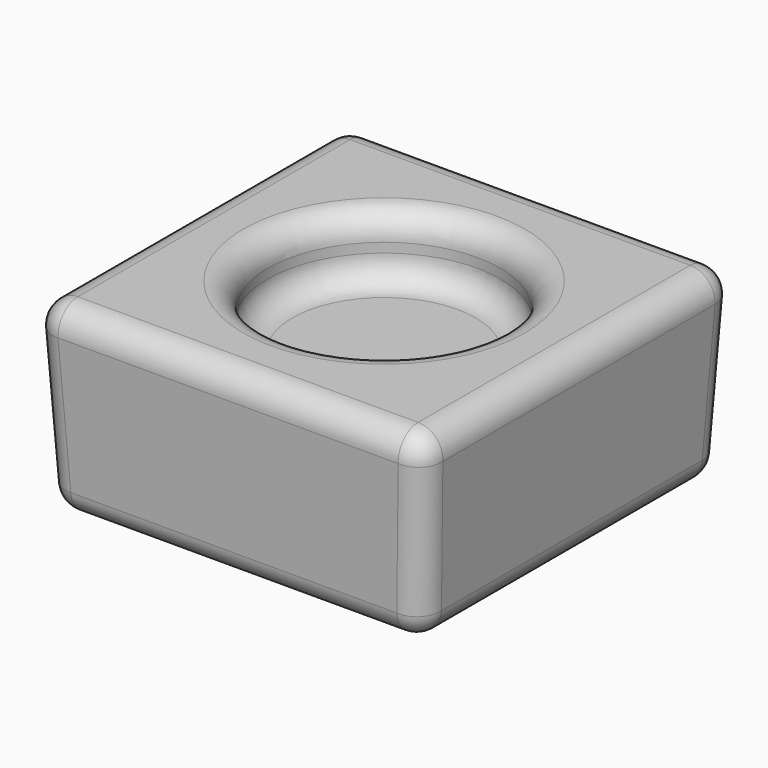
from build123d import *

# Parameters (mm, degrees)
F0_W     = 30
F0_H     = 30
F0_R     = 10
F1_DEPTH = 15
F1_TAPER = -3
F2_DEPTH = 10
F3_R     = 2


with BuildPart() as f1:
    # F0 (on Top) → F1 (new body)
    with BuildSketch(Plane.XY):
        with Locations((-58.3209823817, -55.5250146758)):
            Rectangle(F0_W, F0_H)
        with Locations((-58.3209823817, -55.5250146758)):
            Circle(F0_R, mode=Mode.SUBTRACT)
    extrude(amount=F1_DEPTH, taper=F1_TAPER)

    # F0 (on Top) → F2 (join)
    with BuildSketch(Plane.XY):
        with Locations((-58.3209823817, -55.5250146758)):
            Circle(F0_R)
    extrude(amount=F2_DEPTH)

    # F3
    f3_edges = [f1.edges().sort_by_distance(p)[0] for p in [
        (-67.796905, -55.525015, 10),
        (-67.534866, -55.525015, 15),
        (-42.534866, -55.525015, 15),
        (-58.320982, -39.738898, 15),
        (-58.320982, -71.311131, 15),
        (-74.107099, -55.525015, 15),
        (-58.320982, -40.525015, 0),
        (-73.320982, -55.525015, 0),
        (-58.320982, -70.525015, 0),
        (-43.320982, -55.525015, 0),
        (-42.927924, -70.918073, 7.5),
        (-42.927924, -40.131956, 7.5),
        (-73.714041, -70.918073, 7.5),
        (-73.714041, -40.131956, 7.5),
    ]]
    fillet(f3_edges, radius=F3_R)


solid = f1.part
